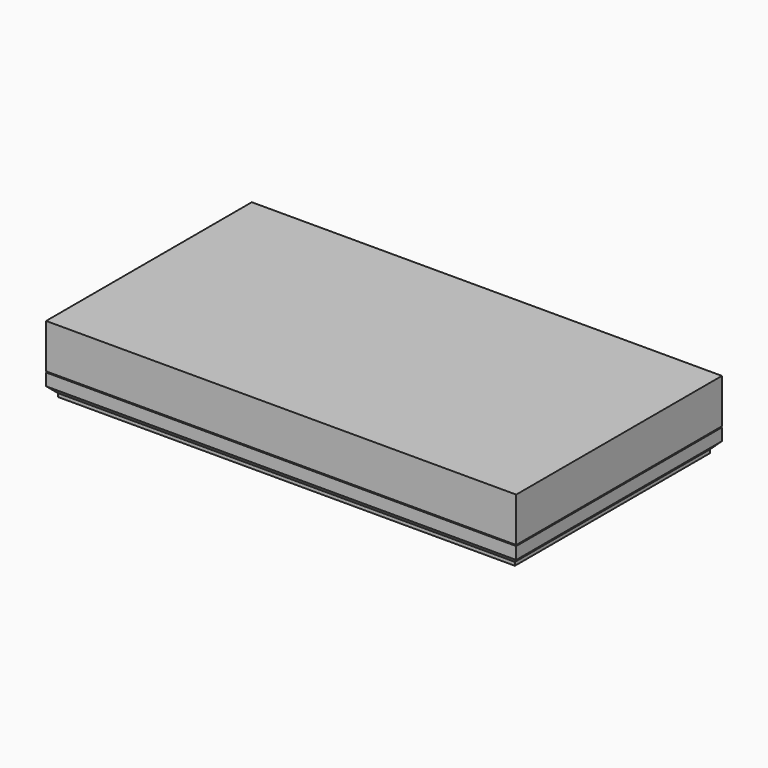
from build123d import *

# Parameters (mm, degrees)
F4_W          = 137.3
F4_H          = 75.1
F5_DEPTH      = 1
F6_W          = 137.3
F6_H          = 75.1
F6_W_2        = 130.3
F6_H_2        = 68.1
F7_DEPTH      = 8.75
F9_DEPTH      = 68.1
F12_W         = 137.3
F12_H         = 75.1
F12_W_2       = 133.5
F12_H_2       = 71.3
F13_DEPTH     = 3.3
F14_W         = 137.3
F14_H         = 75.1
F14_W_2       = 133.5
F14_H_2       = 71.3
F15_DEPTH     = 3
F16_T4_DEPTH  = 133.5
F16_T9_DEPTH  = 71.3
F16_T14_DEPTH = 133.5
F16_T19_DEPTH = 71.3
F16_T25_DEPTH = 138.6433659759
F16_T31_DEPTH = 76.4433659759
F16_T40_DEPTH = 138.6433659759
F16_T46_DEPTH = 76.4433659759
F16_T55_DEPTH = 138.6433659759
F16_T61_DEPTH = 76.4433659759
F16_T70_DEPTH = 76.4433659759
F16_T76_DEPTH = 138.6433659759
F17_W         = 137.3
F17_H         = 75.1
F17_W_2       = 134.1
F17_H_2       = 71.9
F18_DEPTH     = 3.2


# Not quite as in the source:
# - a fillet or chamfer that OpenCascade refuses, or shapes differently, is made with other operations: its cross-section is extruded or revolved along the edge and cut away or added


with BuildPart() as f5:
    # F4 (on Top) → F5 (new body)
    with BuildSketch(Plane.XY):
        Rectangle(F4_W, F4_H)
    extrude(amount=F5_DEPTH)

    # F6 (on face) → F7 (join)
    with BuildSketch(Plane.XY.offset(1)):
        Rectangle(F6_W, F6_H)
        Rectangle(F6_W_2, F6_H_2, mode=Mode.SUBTRACT)
    extrude(amount=F7_DEPTH)

    # F8 (on face) → F9 (join, through all)
    with BuildSketch(Plane.XZ.offset(-34.05)):
        with BuildLine():
            ThreePointArc((-48.25, 9.75), (-56.7, 1.3), (-65.15, 9.75))
            Line((-65.15, 9.75), (-65.15, 1))
            Line((-65.15, 1), (65.15, 1))
            Line((65.15, 1), (65.15, 9.75))
            ThreePointArc((65.15, 9.75), (56.7, 1.3), (48.25, 9.75))
            Line((48.25, 9.75), (46.25, 9.75))
            ThreePointArc((46.25, 9.75), (37.8, 1.3), (29.35, 9.75))
            Line((29.35, 9.75), (27.35, 9.75))
            ThreePointArc((27.35, 9.75), (18.9, 1.3), (10.45, 9.75))
            Line((10.45, 9.75), (8.45, 9.75))
            ThreePointArc((8.45, 9.75), (0, 1.3), (-8.45, 9.75))
            Line((-8.45, 9.75), (-10.45, 9.75))
            ThreePointArc((-10.45, 9.75), (-18.9, 1.3), (-27.35, 9.75))
            Line((-27.35, 9.75), (-29.35, 9.75))
            ThreePointArc((-29.35, 9.75), (-37.8, 1.3), (-46.25, 9.75))
            Line((-46.25, 9.75), (-48.25, 9.75))
        make_face()
    extrude(amount=F9_DEPTH)


with BuildPart() as f11_1:
    # F11: instance of F5
    add(f5.part.mirror(Plane.XY.offset(9.85)))

    # F17 (on face) → F18 (join)
    with BuildSketch(Plane(origin=(0, 0, 9.95), x_dir=(1, 0, 0), z_dir=(0, 0, -1))):
        Rectangle(F17_W, F17_H)
        Rectangle(F17_W_2, F17_H_2, mode=Mode.SUBTRACT)
    extrude(amount=F18_DEPTH)


with BuildPart() as f5_1:
    add(f5.part)

    # F12 (on face) → F13 (cut)
    with BuildSketch(Plane.XY.offset(9.75)):
        Rectangle(F12_W, F12_H)
        Rectangle(F12_W_2, F12_H_2, mode=Mode.SUBTRACT)
    extrude(amount=-F13_DEPTH, mode=Mode.SUBTRACT)

    # F14 (on face) → F15 (cut)
    with BuildSketch(Plane(origin=(0, 0, 0), x_dir=(1, 0, 0), z_dir=(0, 0, -1))):
        Rectangle(F14_W, F14_H)
        Rectangle(F14_W_2, F14_H_2, mode=Mode.SUBTRACT)
    extrude(amount=-F15_DEPTH, mode=Mode.SUBTRACT)

    # F16: chamfer of 2 on 4 edges, made by hand


with BuildPart() as f16_tool2:
    # F16_s3 → F16_t4 (new body)
    with BuildSketch(Plane.YZ.offset(-66.75)):
        Polygon((-37.65, 3), (-35.65, 1), (-35.65, 3), align=None)
    extrude(amount=F16_T4_DEPTH)

    split(bisect_by=Plane.XZ.offset(37.55), keep=Keep.BOTTOM)


with BuildPart() as f5_2:
    add(f5_1.part)

    # F16_t1: union F16_tool2
    add(f16_tool2.part)


with BuildPart() as f16_tool7:
    # F16_s8 → F16_t9 (new body)
    with BuildSketch(Plane.XZ.offset(-35.65)):
        Polygon((-68.75, 3), (-66.75, 1), (-66.75, 3), align=None)
    extrude(amount=F16_T9_DEPTH)

    split(bisect_by=Plane.YZ.offset(-68.65), keep=Keep.TOP)


with BuildPart() as f5_3:
    add(f5_2.part)

    # F16_t6: union F16_tool7
    add(f16_tool7.part)


with BuildPart() as f16_tool12:
    # F16_s13 → F16_t14 (new body)
    with BuildSketch(Plane.YZ.offset(66.75)):
        Polygon((37.65, 3), (35.65, 1), (35.65, 3), align=None)
    extrude(amount=-F16_T14_DEPTH)

    split(bisect_by=Plane.XZ.offset(-37.55), keep=Keep.TOP)


with BuildPart() as f5_4:
    add(f5_3.part)

    # F16_t11: union F16_tool12
    add(f16_tool12.part)


with BuildPart() as f16_tool17:
    # F16_s18 → F16_t19 (new body)
    with BuildSketch(Plane.XZ.offset(35.65)):
        Polygon((68.75, 3), (66.75, 1), (66.75, 3), align=None)
    extrude(amount=-F16_T19_DEPTH)

    split(bisect_by=Plane.YZ.offset(68.65), keep=Keep.BOTTOM)


with BuildPart() as f5_5:
    add(f5_4.part)

    # F16_t16: union F16_tool17
    add(f16_tool17.part)


with BuildPart() as f16_tool23:
    # F16_s24 → F16_t25 (new body)
    with BuildSketch(Plane.YZ.offset(-71.8933659759)):
        Polygon((-37.65, 3), (-35.65, 1), (-35.65, 3), align=None)
    extrude(amount=F16_T25_DEPTH)

    split(bisect_by=Plane.XZ.offset(37.55), keep=Keep.BOTTOM)

    split(bisect_by=Plane.YZ.offset(-68.65), keep=Keep.TOP)

    split(bisect_by=Plane.YZ.offset(-66.75), keep=Keep.BOTTOM)


with BuildPart() as f16_tool29:
    # F16_s30 → F16_t31 (new body)
    with BuildSketch(Plane.XZ.offset(-35.65)):
        Polygon((-68.75, 3), (-66.75, 1), (-66.75, 3), align=None)
    extrude(amount=F16_T31_DEPTH)

    split(bisect_by=Plane.XZ.offset(37.55), keep=Keep.BOTTOM)

    split(bisect_by=Plane.YZ.offset(-68.65), keep=Keep.TOP)

    split(bisect_by=Plane.XZ.offset(35.65), keep=Keep.TOP)


with BuildPart() as f16_tool23_1:
    add(f16_tool23.part)

    # F16_t35: intersect F16_tool29
    add(f16_tool29.part, mode=Mode.INTERSECT)


with BuildPart() as f5_6:
    add(f5_5.part)

    # F16_t21: union F16_tool23
    add(f16_tool23_1.part)


with BuildPart() as f16_tool38:
    # F16_s39 → F16_t40 (new body)
    with BuildSketch(Plane.YZ.offset(-66.75)):
        Polygon((-37.65, 3), (-35.65, 1), (-35.65, 3), align=None)
    extrude(amount=F16_T40_DEPTH)

    split(bisect_by=Plane.XZ.offset(37.55), keep=Keep.BOTTOM)

    split(bisect_by=Plane.YZ.offset(68.65), keep=Keep.BOTTOM)

    split(bisect_by=Plane.YZ.offset(66.75), keep=Keep.TOP)


with BuildPart() as f16_tool44:
    # F16_s45 → F16_t46 (new body)
    with BuildSketch(Plane.XZ.offset(40.7933659759)):
        Polygon((68.75, 3), (66.75, 1), (66.75, 3), align=None)
    extrude(amount=-F16_T46_DEPTH)

    split(bisect_by=Plane.XZ.offset(37.55), keep=Keep.BOTTOM)

    split(bisect_by=Plane.YZ.offset(68.65), keep=Keep.BOTTOM)

    split(bisect_by=Plane.XZ.offset(35.65), keep=Keep.TOP)


with BuildPart() as f16_tool38_1:
    add(f16_tool38.part)

    # F16_t50: intersect F16_tool44
    add(f16_tool44.part, mode=Mode.INTERSECT)


with BuildPart() as f5_7:
    add(f5_6.part)

    # F16_t36: union F16_tool38
    add(f16_tool38_1.part)


with BuildPart() as f16_tool53:
    # F16_s54 → F16_t55 (new body)
    with BuildSketch(Plane.YZ.offset(66.75)):
        Polygon((37.65, 3), (35.65, 1), (35.65, 3), align=None)
    extrude(amount=-F16_T55_DEPTH)

    split(bisect_by=Plane.YZ.offset(-68.65), keep=Keep.TOP)

    split(bisect_by=Plane.XZ.offset(-37.55), keep=Keep.TOP)

    split(bisect_by=Plane.YZ.offset(-66.75), keep=Keep.BOTTOM)


with BuildPart() as f16_tool59:
    # F16_s60 → F16_t61 (new body)
    with BuildSketch(Plane.XZ.offset(-40.7933659759)):
        Polygon((-68.75, 3), (-66.75, 1), (-66.75, 3), align=None)
    extrude(amount=F16_T61_DEPTH)

    split(bisect_by=Plane.YZ.offset(-68.65), keep=Keep.TOP)

    split(bisect_by=Plane.XZ.offset(-37.55), keep=Keep.TOP)

    split(bisect_by=Plane.XZ.offset(-35.65), keep=Keep.BOTTOM)


with BuildPart() as f16_tool53_1:
    add(f16_tool53.part)

    # F16_t65: intersect F16_tool59
    add(f16_tool59.part, mode=Mode.INTERSECT)


with BuildPart() as f5_8:
    add(f5_7.part)

    # F16_t51: union F16_tool53
    add(f16_tool53_1.part)


with BuildPart() as f16_tool68:
    # F16_s69 → F16_t70 (new body)
    with BuildSketch(Plane.XZ.offset(35.65)):
        Polygon((68.75, 3), (66.75, 1), (66.75, 3), align=None)
    extrude(amount=-F16_T70_DEPTH)

    split(bisect_by=Plane.YZ.offset(68.65), keep=Keep.BOTTOM)

    split(bisect_by=Plane.XZ.offset(-37.55), keep=Keep.TOP)

    split(bisect_by=Plane.XZ.offset(-35.65), keep=Keep.BOTTOM)


with BuildPart() as f16_tool74:
    # F16_s75 → F16_t76 (new body)
    with BuildSketch(Plane.YZ.offset(71.8933659759)):
        Polygon((37.65, 3), (35.65, 1), (35.65, 3), align=None)
    extrude(amount=-F16_T76_DEPTH)

    split(bisect_by=Plane.YZ.offset(68.65), keep=Keep.BOTTOM)

    split(bisect_by=Plane.XZ.offset(-37.55), keep=Keep.TOP)

    split(bisect_by=Plane.YZ.offset(66.75), keep=Keep.TOP)


with BuildPart() as f16_tool68_1:
    add(f16_tool68.part)

    # F16_t80: intersect F16_tool74
    add(f16_tool74.part, mode=Mode.INTERSECT)


with BuildPart() as f5_9:
    add(f5_8.part)

    # F16_t66: union F16_tool68
    add(f16_tool68_1.part)


solid = Compound([f11_1.part, f5_9.part])
